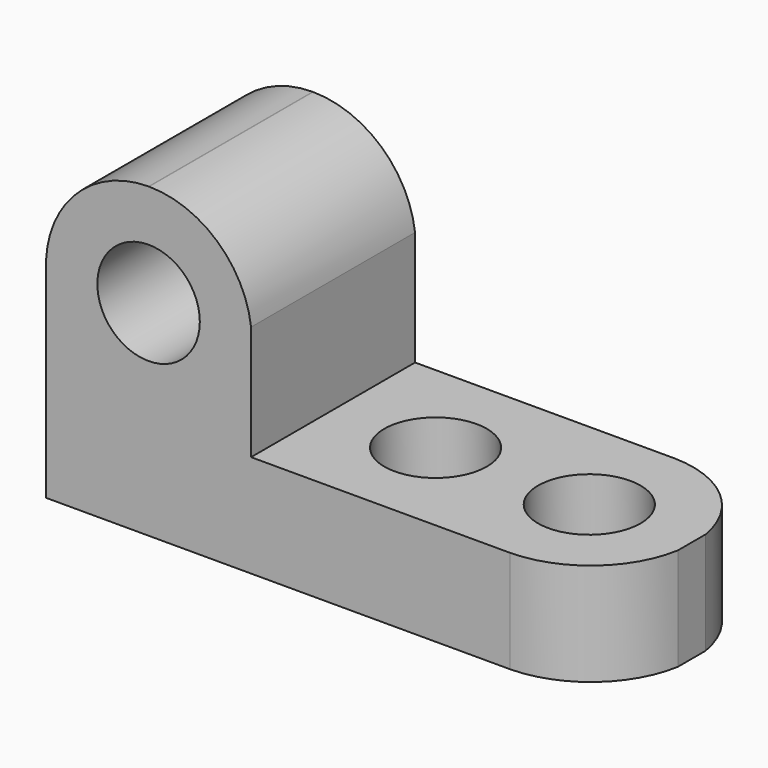
from build123d import *

# Parameters (mm, degrees)
F1_DEPTH = 25.4
F2_R     = 6.35
F3_DEPTH = 25.4
F4_R     = 6.35
F5_DEPTH = 12.7


# Not quite as in the source:
# - ends of sketch curves that miss each other by under 0.0002 mm in the source are joined


with BuildPart() as f1:
    # F0 (on Front) → F1 (new body)
    with BuildSketch(Plane.XZ):
        Polygon((0, 38.1), (0, 0), (69.85, 0), (69.85, 12.7), (25.3999973736, 12.7), (25.3999973736, 38.1), align=None)
    extrude(amount=F1_DEPTH)

    # F2 (on face) → F3 (cut)
    with BuildSketch(Plane.XZ.offset(25.4)):
        with Locations((12.7, 25.4)):
            Circle(F2_R)
        with BuildLine():
            ThreePointArc((12.7392116615, 38.1000602784), (21.1944094362, 34.8947951162), (25.3999973736, 26.8899763006))
            Line((25.3999973736, 26.8899763006), (25.3999973736, 38.1))
            Line((25.3999973736, 38.1), (12.7392116615, 38.1000602784))
        make_face()
        with BuildLine():
            ThreePointArc((0, 25.9728431702), (3.9449392563, 34.5834780061), (12.7392116615, 38.1000602784))
            Line((12.7392116615, 38.1000602784), (0, 38.1))
            Line((0, 38.1), (0, 25.9728431702))
        make_face()
    extrude(amount=-F3_DEPTH, mode=Mode.SUBTRACT)

    # F4 (on face) → F5 (cut)
    with BuildSketch(Plane.XY.offset(12.7)):
        with Locations((38.1, -12.7)):
            Circle(F4_R)
        with Locations((57.15, -12.7)):
            Circle(F4_R)
        with BuildLine():
            ThreePointArc((57.5116686145, 0), (65.5882036204, -3.0491682704), (69.85, -10.5568267911))
            Line((69.85, -10.5568267911), (69.85, 0))
            Line((69.85, 0), (57.5116686145, 0))
        make_face()
        with BuildLine():
            ThreePointArc((69.85, -14.8431732089), (65.5882036204, -22.3508317296), (57.5116686145, -25.4))
            Line((57.5116686145, -25.4), (69.85, -25.4))
            Line((69.85, -25.4), (69.85, -14.8431732089))
        make_face()
    extrude(amount=-F5_DEPTH, mode=Mode.SUBTRACT)


solid = f1.part
